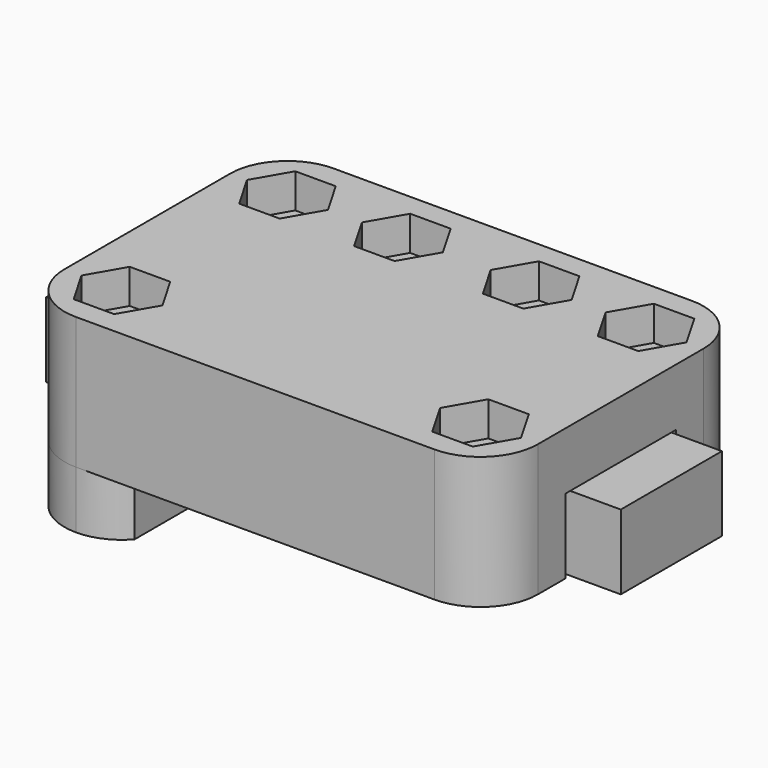
from build123d import *

# Parameters (mm, degrees)
F0_W     = 50
F0_H     = 11
F1_DEPTH = 6.5
F2_R     = 1.5
F3_DEPTH = 6.5
F4_R     = 1.5
F5_DEPTH = 5
F6_R     = 1.5
F7_DEPTH = 5
F9_DEPTH = 3


with BuildPart() as f1:
    # F0 (on Top) → F1 (new body)
    with BuildSketch(Plane.XY):
        Rectangle(F0_W, F0_H)
    extrude(amount=F1_DEPTH)


with BuildPart() as f3:
    # F2 (on Top) → F3 (new body)
    with BuildSketch(Plane.XY):
        with BuildLine():
            Line((15.6, 14), (0, 14))
            Line((0, 14), (-15.6, 14))
            ThreePointArc((-15.6, 14), (-19.1355339059, 12.5355339059), (-20.6, 9))
            Line((-20.6, 9), (-20.6, 6))
            Line((-20.6, 6), (0, 6))
            Line((0, 6), (20.6, 6))
            Line((20.6, 6), (20.6, 9))
            ThreePointArc((20.6, 9), (19.1355339059, 12.5355339059), (15.6, 14))
        make_face()
        with Locations((-15.6, 9)):
            Circle(F2_R, mode=Mode.SUBTRACT)
        with Locations((-5.6, 9)):
            Circle(F2_R, mode=Mode.SUBTRACT)
        with Locations((5.6, 9)):
            Circle(F2_R, mode=Mode.SUBTRACT)
        with Locations((15.6, 9)):
            Circle(F2_R, mode=Mode.SUBTRACT)
    extrude(amount=F3_DEPTH)



with BuildPart() as f3b:
    # F2 (on Top) → F3, piece 2 (new body)
    with BuildSketch(Plane.XY):
        with BuildLine():
            Line((0, -6), (-20.6, -6))
            Line((-20.6, -6), (-20.6, -9))
            ThreePointArc((-20.6, -9), (-19.1355339059, -12.5355339059), (-15.6, -14))
            Line((-15.6, -14), (0, -14))
            Line((0, -14), (15.6, -14))
            ThreePointArc((15.6, -14), (19.1355339059, -12.5355339059), (20.6, -9))
            Line((20.6, -9), (20.6, -6))
            Line((20.6, -6), (0, -6))
        make_face()
        with Locations((-15.6, -9)):
            Circle(F2_R, mode=Mode.SUBTRACT)
        with Locations((15.6, -9)):
            Circle(F2_R, mode=Mode.SUBTRACT)
    extrude(amount=F3_DEPTH)


with BuildPart() as f3_1:
    add(f3.part)

    add(f3b.part)  # F5 merges F3b
    # F4 (on face) → F5 (join)
    with BuildSketch(Plane.XY.offset(6.5)):
        with BuildLine():
            Line((15.6, 14), (0, 14))
            Line((0, 14), (-15.6, 14))
            ThreePointArc((-15.6, 14), (-19.1355339059, 12.5355339059), (-20.6, 9))
            Line((-20.6, 9), (-20.6, -9))
            ThreePointArc((-20.6, -9), (-19.1355339059, -12.5355339059), (-15.6, -14))
            Line((-15.6, -14), (0, -14))
            Line((0, -14), (15.6, -14))
            ThreePointArc((15.6, -14), (19.1355339059, -12.5355339059), (20.6, -9))
            Line((20.6, -9), (20.6, 9))
            ThreePointArc((20.6, 9), (19.1355339059, 12.5355339059), (15.6, 14))
        make_face()
        with Locations((-15.6, -9)):
            Circle(F4_R, mode=Mode.SUBTRACT)
        with Locations((15.6, -9)):
            Circle(F4_R, mode=Mode.SUBTRACT)
        with Locations((-15.6, 9)):
            Circle(F4_R, mode=Mode.SUBTRACT)
        with Locations((-5.6, 9)):
            Circle(F4_R, mode=Mode.SUBTRACT)
        with Locations((5.6, 9)):
            Circle(F4_R, mode=Mode.SUBTRACT)
        with Locations((15.6, 9)):
            Circle(F4_R, mode=Mode.SUBTRACT)
    extrude(amount=F5_DEPTH)

    # F8 (on face) → F9 (cut)
    with BuildSketch(Plane.XY.offset(11.5)):
        Polygon((-13.839081679, 12.05), (-17.360918321, 12.05), (-19.1218366421, 9), (-17.360918321, 5.95), (-13.839081679, 5.95), (-12.0781633579, 9), align=None)
        Polygon((17.360918321, 5.95), (19.1218366421, 9), (17.360918321, 12.05), (13.839081679, 12.05), (12.0781633579, 9), (13.839081679, 5.95), align=None)
        Polygon((-19.1218366421, -9), (-17.360918321, -12.05), (-13.839081679, -12.05), (-12.0781633579, -9), (-13.839081679, -5.95), (-17.360918321, -5.95), align=None)
        Polygon((13.839081679, -12.05), (17.360918321, -12.05), (19.1218366421, -9), (17.360918321, -5.95), (13.839081679, -5.95), (12.0781633579, -9), align=None)
        Polygon((-2.0781633579, 9), (-3.839081679, 12.05), (-7.360918321, 12.05), (-9.1218366421, 9), (-7.360918321, 5.95), (-3.839081679, 5.95), align=None)
        Polygon((3.839081679, 5.95), (7.360918321, 5.95), (9.1218366421, 9), (7.360918321, 12.05), (3.839081679, 12.05), (2.0781633579, 9), align=None)
    extrude(amount=-F9_DEPTH, mode=Mode.SUBTRACT)


with BuildPart() as f7:
    # F6 (on face) → F7 (new body)
    with BuildSketch(Plane(origin=(0, 0, 0), x_dir=(1, 0, 0), z_dir=(0, 0, -1))):
        with BuildLine():
            ThreePointArc((-15.6, 14), (-19.1355339059, 12.5355339059), (-20.6, 9))
            Line((-20.6, 9), (-20.6, 0))
            Line((-20.6, 0), (-20.6, -9))
            ThreePointArc((-20.6, -9), (-19.1355339059, -12.5355339059), (-15.6, -14))
            ThreePointArc((-15.6, -14), (-13.5428108612, -13.5571891388), (-11.85, -12.3071891388))
            Line((-11.85, -12.3071891388), (-11.85, 9))
            Line((-11.85, 9), (-11.85, 12.3071891388))
            ThreePointArc((-11.85, 12.3071891388), (-13.5428108612, 13.5571891388), (-15.6, 14))
        make_face()
        with Locations((-15.6, -9)):
            Circle(F6_R, mode=Mode.SUBTRACT)
        with Locations((-15.6, 9)):
            Circle(F6_R, mode=Mode.SUBTRACT)
    extrude(amount=F7_DEPTH)


solid = Compound([f1.part, f3_1.part, f7.part])
